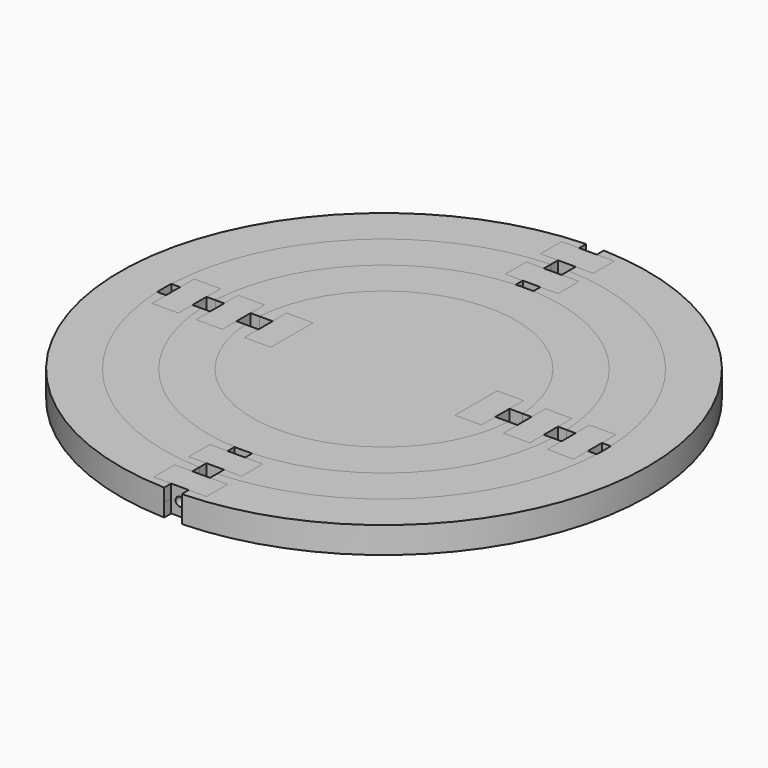
from build123d import *

# Parameters (mm, degrees)
F2_DEPTH      = 1.5
F2_DEPTH_BACK = 1.5
F3_DEPTH      = 1.5
F3_DEPTH_BACK = 1.5
F4_DEPTH      = 1.5
F4_DEPTH_BACK = 1.5
F5_DEPTH      = 1.5
F5_DEPTH_BACK = 1.5
F6_W          = 4
F6_H          = 3
F6_W_2        = 2
F6_W_3        = 6
F6_W_4        = 3
F6_H_2        = 6
F6_H_3        = 2
F7_DEPTH      = 3.001
F8_DEPTH      = 3
F9_R          = 0.5
F10_DEPTH     = 58.9659890485
F11_R         = 0.5
F12_DEPTH     = 53.9784881745


# Not quite as in the source:
# - a feature of the source that left no trace in its solid (it failed there, or was rolled back) is left out


with BuildPart() as f2:
    # F1 (on Top) → F2 (new body, two sides)
    with BuildSketch(Plane.XY) as f2_sk:
        with BuildLine():
            Line((-1, 24.9799919936), (-1, 29.9833287011))
            ThreePointArc((-1, 29.9833287011), (-30, 0), (-1, -29.9833287011))
            Line((-1, -29.9833287011), (-1, -24.9799919936))
            ThreePointArc((-1, -24.9799919936), (-17.6776695297, -17.6776695297), (-24.9799919936, -1))
            ThreePointArc((-24.9799919936, -1), (-25, 0), (-24.9799919936, 1))
            ThreePointArc((-24.9799919936, 1), (-17.6776695297, 17.6776695297), (-1, 24.9799919936))
        make_face()
    extrude(amount=F2_DEPTH)
    extrude(f2_sk.sketch, amount=-F2_DEPTH_BACK)


with BuildPart() as f2b:
    # F1 (on Top) → F2, piece 2 (new body, two sides)
    with BuildSketch(Plane.XY) as f2_2_sk:
        with BuildLine():
            ThreePointArc((1, -29.9833287011), (21.5638586528, -20.8566536146), (30, 0))
            ThreePointArc((30, 0), (21.5638586528, 20.8566536146), (1, 29.9833287011))
            Line((1, 29.9833287011), (1, 24.9799919936))
            ThreePointArc((1, 24.9799919936), (17.6776695297, 17.6776695297), (24.9799919936, 1))
            ThreePointArc((24.9799919936, 1), (24.9949974979, 0.5001000701), (25, 0))
            ThreePointArc((25, 0), (24.9949974979, -0.5001000701), (24.9799919936, -1))
            ThreePointArc((24.9799919936, -1), (17.6776695297, -17.6776695297), (1, -24.9799919936))
            Line((1, -24.9799919936), (1, -29.9833287011))
        make_face()
    extrude(amount=F2_DEPTH)
    extrude(f2_2_sk.sketch, amount=-F2_DEPTH_BACK)


with BuildPart() as f3:
    # F1 (on Top) → F3 (new body, two sides)
    with BuildSketch(Plane.XY) as f3_sk:
        with BuildLine():
            Line((-1, 19.9749843554), (-1, 24.9799919936))
            ThreePointArc((-1, 24.9799919936), (-17.6776695297, 17.6776695297), (-24.9799919936, 1))
            Line((-24.9799919936, 1), (-19.9749843554, 1))
            ThreePointArc((-19.9749843554, 1), (-14.1421356237, 14.1421356237), (-1, 19.9749843554))
        make_face()
    extrude(amount=F3_DEPTH)
    extrude(f3_sk.sketch, amount=-F3_DEPTH_BACK)


with BuildPart() as f3b:
    # F1 (on Top) → F3, piece 2 (new body, two sides)
    with BuildSketch(Plane.XY) as f3_2_sk:
        with BuildLine():
            ThreePointArc((-24.9799919936, -1), (-17.6776695297, -17.6776695297), (-1, -24.9799919936))
            Line((-1, -24.9799919936), (-1, -19.9749843554))
            ThreePointArc((-1, -19.9749843554), (-14.1421356237, -14.1421356237), (-19.9749843554, -1))
            Line((-19.9749843554, -1), (-24.9799919936, -1))
        make_face()
    extrude(amount=F3_DEPTH)
    extrude(f3_2_sk.sketch, amount=-F3_DEPTH_BACK)


with BuildPart() as f3c:
    # F1 (on Top) → F3, piece 3 (new body, two sides)
    with BuildSketch(Plane.XY) as f3_3_sk:
        with BuildLine():
            Line((1, -19.9749843554), (1, -24.9799919936))
            ThreePointArc((1, -24.9799919936), (17.6776695297, -17.6776695297), (24.9799919936, -1))
            Line((24.9799919936, -1), (19.9749843554, -1))
            ThreePointArc((19.9749843554, -1), (14.1421356237, -14.1421356237), (1, -19.9749843554))
        make_face()
    extrude(amount=F3_DEPTH)
    extrude(f3_3_sk.sketch, amount=-F3_DEPTH_BACK)


with BuildPart() as f3d:
    # F1 (on Top) → F3, piece 4 (new body, two sides)
    with BuildSketch(Plane.XY) as f3_4_sk:
        with BuildLine():
            ThreePointArc((24.9799919936, 1), (17.6776695297, 17.6776695297), (1, 24.9799919936))
            Line((1, 24.9799919936), (1, 19.9749843554))
            ThreePointArc((1, 19.9749843554), (14.1421356237, 14.1421356237), (19.9749843554, 1))
            Line((19.9749843554, 1), (24.9799919936, 1))
        make_face()
    extrude(amount=F3_DEPTH)
    extrude(f3_4_sk.sketch, amount=-F3_DEPTH_BACK)


with BuildPart() as f4:
    # F1 (on Top) → F4 (new body, two sides)
    with BuildSketch(Plane.XY) as f4_sk:
        with BuildLine():
            ThreePointArc((19.9749843554, 1), (14.1421356237, 14.1421356237), (1, 19.9749843554))
            ThreePointArc((1, 19.9749843554), (0, 20), (-1, 19.9749843554))
            ThreePointArc((-1, 19.9749843554), (-14.1421356237, 14.1421356237), (-19.9749843554, 1))
            Line((-19.9749843554, 1), (-14.9666295471, 1))
            ThreePointArc((-14.9666295471, 1), (0, 15), (14.9666295471, 1))
            Line((14.9666295471, 1), (19.9749843554, 1))
        make_face()
    extrude(amount=F4_DEPTH)
    extrude(f4_sk.sketch, amount=-F4_DEPTH_BACK)


with BuildPart() as f4b:
    # F1 (on Top) → F4, piece 2 (new body, two sides)
    with BuildSketch(Plane.XY) as f4_2_sk:
        with BuildLine():
            ThreePointArc((-1, -19.9749843554), (0, -20), (1, -19.9749843554))
            ThreePointArc((1, -19.9749843554), (14.1421356237, -14.1421356237), (19.9749843554, -1))
            Line((19.9749843554, -1), (14.9666295471, -1))
            ThreePointArc((14.9666295471, -1), (0, -15), (-14.9666295471, -1))
            Line((-14.9666295471, -1), (-19.9749843554, -1))
            ThreePointArc((-19.9749843554, -1), (-14.1421356237, -14.1421356237), (-1, -19.9749843554))
        make_face()
    extrude(amount=F4_DEPTH)
    extrude(f4_2_sk.sketch, amount=-F4_DEPTH_BACK)


with BuildPart() as f5:
    # F1 (on Top) → F5 (new body, two sides)
    with BuildSketch(Plane.XY) as f5_sk:
        with BuildLine():
            ThreePointArc((15, 0), (14.9916550655, 0.5002783193), (14.9666295471, 1))
            ThreePointArc((14.9666295471, 1), (0, 15), (-14.9666295471, 1))
            ThreePointArc((-14.9666295471, 1), (-15, 0), (-14.9666295471, -1))
            ThreePointArc((-14.9666295471, -1), (0, -15), (14.9666295471, -1))
            ThreePointArc((14.9666295471, -1), (14.9916550655, -0.5002783193), (15, 0))
        make_face()
    extrude(amount=F5_DEPTH)
    extrude(f5_sk.sketch, amount=-F5_DEPTH_BACK)


with BuildPart() as f7_tool:
    # F6 (on face) → F7 (new body, through all)
    with BuildSketch(Plane.XY.offset(1.5)):
        with Locations((1, 27.4816603474)):
            Rectangle(F6_W, F6_H)
        with Locations((-2, 27.4816603474)):
            Rectangle(F6_W_2, F6_H)
        with Locations((1, -27.4816603474)):
            Rectangle(F6_W, F6_H)
        with Locations((-2, -27.4816603474)):
            Rectangle(F6_W_2, F6_H)
        with Locations((0, -22.4774881745)):
            Rectangle(F6_W_3, F6_H)
        with Locations((0, 22.4774881745)):
            Rectangle(F6_W_3, F6_H)
        Polygon((18.9708069513, -3), (18.9708069513, 3), (15.9708069513, 3), (15.9708069513, 1), (15.9708069513, -1), (15.9708069513, -3), align=None)
        with Locations((22.4774881745, 0)):
            Rectangle(F6_W_4, F6_H_2)
        with Locations((-22.4774881745, -2)):
            Rectangle(F6_W_4, F6_H_3)
        with Locations((-22.4774881745, 0)):
            Rectangle(F6_W_4, F6_H_3)
        with Locations((-22.4774881745, 2)):
            Rectangle(F6_W_4, F6_H_3)
        with Locations((-17.4708069513, 2)):
            Rectangle(F6_W_4, F6_H_3)
        with Locations((-17.4708069513, 0)):
            Rectangle(F6_W_4, F6_H_3)
        with Locations((-17.4708069513, -2)):
            Rectangle(F6_W_4, F6_H_3)
        Polygon((-14.9666295471, 1), (-15.9708069513, 1), (-15.9708069513, -1), (-14.9666295471, -1), (-13.4666295471, -1), (-13.4666295471, 1), align=None)
        Polygon((-13.4666295471, 3), (-13.4666295471, 1), (-13.4666295471, -1), (-13.4666295471, -3), (-10.4666295471, -3), (-10.4666295471, 3), align=None)
        Polygon((13.4666295471, -1), (13.4666295471, 1), (13.4666295471, 3), (10.4666295471, 3), (10.4666295471, -3), (13.4666295471, -3), align=None)
        Polygon((15.9708069513, -1), (15.9708069513, 1), (14.9666295471, 1), (13.4666295471, 1), (13.4666295471, -1), (14.9666295471, -1), align=None)
    extrude(amount=-F7_DEPTH)


with BuildPart() as f2_1:
    add(f2.part)

    # F7: cut by f7_tool
    add(f7_tool.part, mode=Mode.SUBTRACT)


with BuildPart() as f2b_1:
    add(f2b.part)

    # F7: cut by f7_tool
    add(f7_tool.part, mode=Mode.SUBTRACT)


with BuildPart() as f3_1:
    add(f3.part)

    # F7: cut by f7_tool
    add(f7_tool.part, mode=Mode.SUBTRACT)


with BuildPart() as f3b_1:
    add(f3b.part)

    # F7: cut by f7_tool
    add(f7_tool.part, mode=Mode.SUBTRACT)


with BuildPart() as f3c_1:
    add(f3c.part)

    # F7: cut by f7_tool
    add(f7_tool.part, mode=Mode.SUBTRACT)


with BuildPart() as f3d_1:
    add(f3d.part)

    # F7: cut by f7_tool
    add(f7_tool.part, mode=Mode.SUBTRACT)


with BuildPart() as f4_1:
    add(f4.part)

    # F7: cut by f7_tool
    add(f7_tool.part, mode=Mode.SUBTRACT)


with BuildPart() as f4b_1:
    add(f4b.part)

    # F7: cut by f7_tool
    add(f7_tool.part, mode=Mode.SUBTRACT)


with BuildPart() as f5_1:
    add(f5.part)

    # F7: cut by f7_tool
    add(f7_tool.part, mode=Mode.SUBTRACT)


with BuildPart() as f8:
    # F6 (on face) → F8 (new body)
    with BuildSketch(Plane.XY.offset(1.5)):
        with Locations((-2, 27.4816603474)):
            Rectangle(F6_W_2, F6_H)
        with Locations((1, 27.4816603474)):
            Rectangle(F6_W, F6_H)
    extrude(amount=-F8_DEPTH)


with BuildPart() as f8b:
    # F6 (on face) → F8, piece 2 (new body)
    with BuildSketch(Plane.XY.offset(1.5)):
        with Locations((0, 22.4774881745)):
            Rectangle(F6_W_3, F6_H)
    extrude(amount=-F8_DEPTH)


with BuildPart() as f8c:
    # F6 (on face) → F8, piece 3 (new body)
    with BuildSketch(Plane.XY.offset(1.5)):
        with Locations((1, -27.4816603474)):
            Rectangle(F6_W, F6_H)
        with Locations((-2, -27.4816603474)):
            Rectangle(F6_W_2, F6_H)
    extrude(amount=-F8_DEPTH)


with BuildPart() as f8d:
    # F6 (on face) → F8, piece 4 (new body)
    with BuildSketch(Plane.XY.offset(1.5)):
        with Locations((0, -22.4774881745)):
            Rectangle(F6_W_3, F6_H)
    extrude(amount=-F8_DEPTH)


with BuildPart() as f8e:
    # F6 (on face) → F8, piece 5 (new body)
    with BuildSketch(Plane.XY.offset(1.5)):
        with Locations((-22.4774881745, 2)):
            Rectangle(F6_W_4, F6_H_3)
        with Locations((-22.4774881745, 0)):
            Rectangle(F6_W_4, F6_H_3)
        with Locations((-22.4774881745, -2)):
            Rectangle(F6_W_4, F6_H_3)
    extrude(amount=-F8_DEPTH)


with BuildPart() as f8f:
    # F6 (on face) → F8, piece 6 (new body)
    with BuildSketch(Plane.XY.offset(1.5)):
        with Locations((-17.4708069513, 2)):
            Rectangle(F6_W_4, F6_H_3)
        with Locations((-17.4708069513, 0)):
            Rectangle(F6_W_4, F6_H_3)
        with Locations((-17.4708069513, -2)):
            Rectangle(F6_W_4, F6_H_3)
    extrude(amount=-F8_DEPTH)


with BuildPart() as f8g:
    # F6 (on face) → F8, piece 7 (new body)
    with BuildSketch(Plane.XY.offset(1.5)):
        Polygon((18.9708069513, -3), (18.9708069513, 3), (15.9708069513, 3), (15.9708069513, 1), (15.9708069513, -1), (15.9708069513, -3), align=None)
    extrude(amount=-F8_DEPTH)


with BuildPart() as f8h:
    # F6 (on face) → F8, piece 8 (new body)
    with BuildSketch(Plane.XY.offset(1.5)):
        with Locations((22.4774881745, 0)):
            Rectangle(F6_W_4, F6_H_2)
    extrude(amount=-F8_DEPTH)


with BuildPart() as f8i:
    # F6 (on face) → F8, piece 9 (new body)
    with BuildSketch(Plane.XY.offset(1.5)):
        Polygon((-13.4666295471, 3), (-13.4666295471, 1), (-13.4666295471, -1), (-13.4666295471, -3), (-10.4666295471, -3), (-10.4666295471, 3), align=None)
    extrude(amount=-F8_DEPTH)


with BuildPart() as f8j:
    # F6 (on face) → F8, piece 10 (new body)
    with BuildSketch(Plane.XY.offset(1.5)):
        Polygon((13.4666295471, -1), (13.4666295471, 1), (13.4666295471, 3), (10.4666295471, 3), (10.4666295471, -3), (13.4666295471, -3), align=None)
    extrude(amount=-F8_DEPTH)


with BuildPart() as f10_tool:
    # F9 (on face) → F10 (new body, through all)
    with BuildSketch(Plane(origin=(0, 28.9816603474, 0), x_dir=(-1, 0, 0), z_dir=(0, 1, 0))):
        Circle(F9_R)
    extrude(amount=-F10_DEPTH)


with BuildPart() as f8_1:
    add(f8.part)

    # F10: cut by f10_tool
    add(f10_tool.part, mode=Mode.SUBTRACT)


with BuildPart() as f8b_1:
    add(f8b.part)

    # F10: cut by f10_tool
    add(f10_tool.part, mode=Mode.SUBTRACT)


with BuildPart() as f8c_1:
    add(f8c.part)

    # F10: cut by f10_tool
    add(f10_tool.part, mode=Mode.SUBTRACT)


with BuildPart() as f8d_1:
    add(f8d.part)

    # F10: cut by f10_tool
    add(f10_tool.part, mode=Mode.SUBTRACT)


with BuildPart() as f12_tool:
    # F11 (on face) → F12 (new body, through all)
    with BuildSketch(Plane(origin=(-23.9774881745, 0, 0), x_dir=(0, -1, 0), z_dir=(-1, 0, 0))):
        Circle(F11_R)
    extrude(amount=-F12_DEPTH)


with BuildPart() as f8e_1:
    add(f8e.part)

    # F12: cut by f12_tool
    add(f12_tool.part, mode=Mode.SUBTRACT)


with BuildPart() as f8f_1:
    add(f8f.part)

    # F12: cut by f12_tool
    add(f12_tool.part, mode=Mode.SUBTRACT)


with BuildPart() as f8g_1:
    add(f8g.part)

    # F12: cut by f12_tool
    add(f12_tool.part, mode=Mode.SUBTRACT)


with BuildPart() as f8h_1:
    add(f8h.part)

    # F12: cut by f12_tool
    add(f12_tool.part, mode=Mode.SUBTRACT)


with BuildPart() as f8i_1:
    add(f8i.part)

    # F12: cut by f12_tool
    add(f12_tool.part, mode=Mode.SUBTRACT)


with BuildPart() as f8j_1:
    add(f8j.part)

    # F12: cut by f12_tool
    add(f12_tool.part, mode=Mode.SUBTRACT)


solid = Compound([f2_1.part, f2b_1.part, f3_1.part, f3b_1.part, f3c_1.part, f3d_1.part, f4_1.part, f4b_1.part, f5_1.part, f8_1.part, f8b_1.part, f8c_1.part, f8d_1.part, f8e_1.part, f8f_1.part, f8g_1.part, f8h_1.part, f8i_1.part, f8j_1.part])
